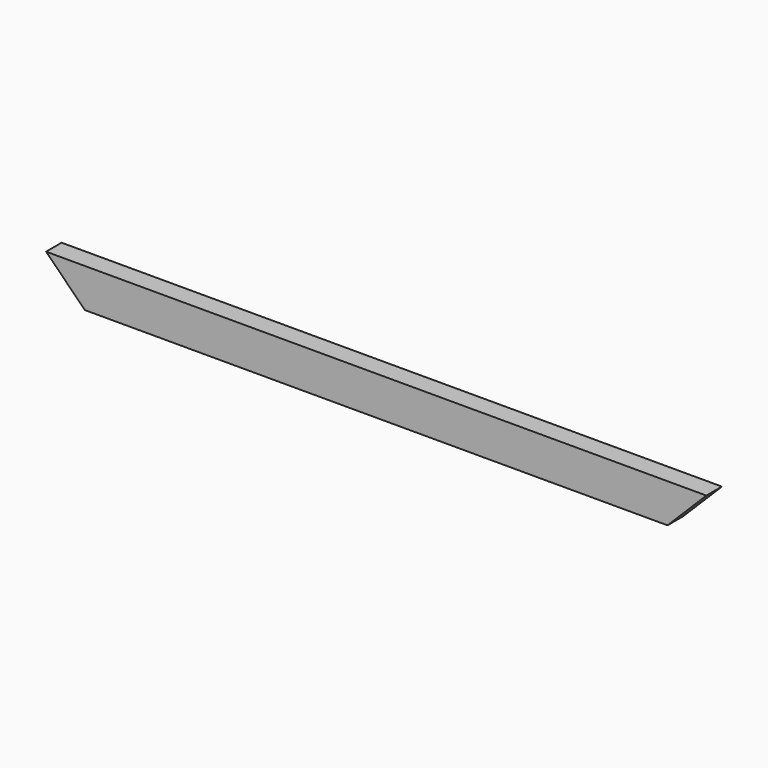
from build123d import *

# Parameters (mm, degrees)
F0_W     = 340
F0_H     = 20
F1_DEPTH = 10
F2_SIZE  = 19.99999


# Not quite as in the source:
# - a fillet or chamfer is up to 0.001 mm smaller than in the source, because OpenCascade refuses the exact size


with BuildPart() as f1:
    # F0 (on Front) → F1 (new body)
    with BuildSketch(Plane.XZ):
        with Locations((109.6177828312, 37.3797959089)):
            Rectangle(F0_W, F0_H)
    extrude(amount=F1_DEPTH)

    # F2 (size 20 in the source; OpenCascade refuses exactly that, so slightly less here)
    f2_edges = [f1.edges().sort_by_distance(p)[0] for p in [
        (-60.382217, -5, 27.379796),
        (279.617783, -5, 27.379796),
    ]]
    chamfer(f2_edges, length=F2_SIZE)


solid = f1.part
